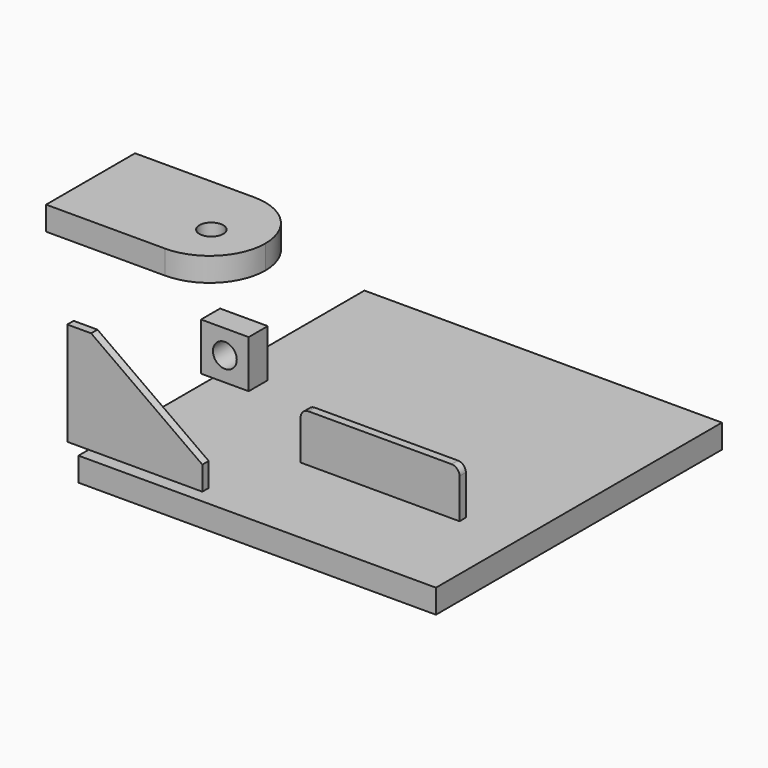
from build123d import *

# Parameters (mm, degrees)
F1_DEPTH  = 6.35
F0_W      = 127
F0_H      = 38.1
F2_R      = 6.35
F3_W      = 285.75
F3_H      = 19.05
F4_DEPTH  = 285.75
F5_W      = 38.1
F5_H      = 38.1
F5_R      = 9.525
F6_DEPTH  = 19.05
F7_W      = 139.7
F7_H      = 19.05
F8_DEPTH  = 88.9
F9_R      = 9.525
F10_DEPTH = 50.8
F11_R     = 44.44999


# Not quite as in the source:
# - a fillet or chamfer is up to 0.001 mm smaller than in the source, because OpenCascade refuses the exact size


with BuildPart() as f1:
    # F0 (on Front) → F1 (new body)
    with BuildSketch(Plane.XZ):
        Polygon((-28.7604803375, 36.4999751758), (-47.8104803375, 36.4999751758), (-47.8104803375, -46.0500248242), (60.1395196625, -46.0500248242), (60.1395196625, -27.0000248242), align=None)
    extrude(amount=F1_DEPTH)


with BuildPart() as f1b:
    # F0 (on Front) → F1, piece 2 (new body)
    with BuildSketch(Plane.XZ):
        with Locations((202.2152820826, 19.05)):
            Rectangle(F0_W, F0_H)
    extrude(amount=F1_DEPTH)

    # F2
    f2_edges = [f1b.edges().sort_by_distance(p)[0] for p in [
        (138.715282, -3.175, 38.1),
        (265.715282, -3.175, 38.1),
    ]]
    fillet(f2_edges, radius=F2_R)


with BuildPart() as f4:
    # F3 (on Front) → F4 (new body)
    with BuildSketch(Plane.XZ):
        with Locations((98.9142842591, -66.6212261169)):
            Rectangle(F3_W, F3_H)
    extrude(amount=-F4_DEPTH)


with BuildPart() as f6:
    # F5 (on Front) → F6 (new body)
    with BuildSketch(Plane.XZ):
        with Locations((88.29173321, 64.1970857978)):
            Rectangle(F5_W, F5_H)
        with Locations((88.29173321, 64.1970857978)):
            Circle(F5_R, mode=Mode.SUBTRACT)
    extrude(amount=F6_DEPTH)


with BuildPart() as f8:
    # F7 (on Front) → F8 (new body)
    with BuildSketch(Plane.XZ):
        with Locations((0, 101.5910909008)):
            Rectangle(F7_W, F7_H)
    extrude(amount=-F8_DEPTH)

    # F9 (on face) → F10 (cut)
    with BuildSketch(Plane.XY.offset(111.1160909008)):
        with Locations((31.75, 38.1)):
            Circle(F9_R)
    extrude(amount=-F10_DEPTH, mode=Mode.SUBTRACT)

    # F11 (radius 44.45 in the source; OpenCascade refuses exactly that, so slightly less here)
    f11_edges = [f8.edges().sort_by_distance(p)[0] for p in [
        (69.85, 0, 101.591091),
        (69.85, 88.9, 101.591091),
    ]]
    fillet(f11_edges, radius=F11_R)


solid = Compound([f1.part, f1b.part, f4.part, f6.part, f8.part])
